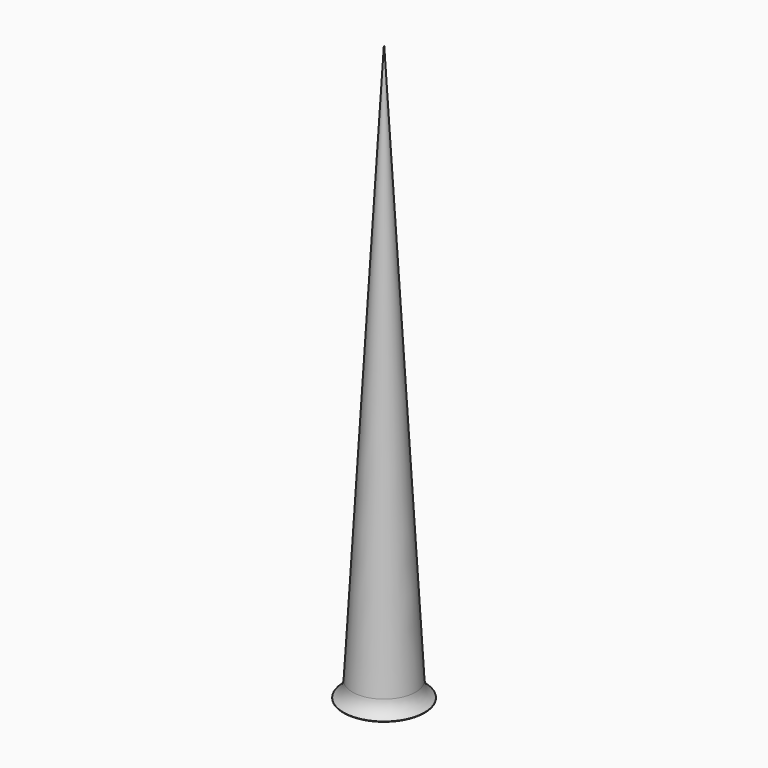
from build123d import *

# Parameters (mm, degrees)
F0_R     = 85
F2_R     = 0.5
F4_R     = 105.9677495378
F5_DEPTH = 1


# Not quite as in the source:
# - a fillet or chamfer that OpenCascade refuses, or shapes differently, is made with other operations: its cross-section is extruded or revolved along the edge and cut away or added


with BuildPart() as f3:
    # F0 (on Top) → F3 section 0
    with BuildSketch(Plane.XY):
        Circle(F0_R)
    # F2 (on offset) → F3 section 1
    with BuildSketch(Plane.XY.offset(1500)):
        Circle(F2_R)
    loft()

    # F4 (on Top) → F5 (join)
    with BuildSketch(Plane.XY):
        Circle(F4_R)
    extrude(amount=F5_DEPTH)

    # F6: fillet of radius 50 on 1 edges, made by hand


with BuildPart() as f6_tool2:
    # F6_s3 → F6_t4 (revolve)
    with BuildSketch(Plane.XZ):
        with BuildLine():
            ThreePointArc((105.9675361519, 0.9996616711), (89.555381413, 17.9202187852), (82.7192415892, 40.4797238448))
            Line((82.7192415892, 40.4797238448), (77.7270102291, 40.1984948115))
            ThreePointArc((77.7270102291, 40.1984948115), (78.8394224512, 20.458644138), (79.9514353065, 0.7187709667))
            Line((79.9514353065, 0.7187709667), (84.9436666667, -4.0001463701))
            ThreePointArc((84.9436666667, -4.0001463701), (95.4556014093, -4.0001463701), (103.300134248, -3.2295735796))
            Line((103.300134248, -3.2295735796), (105.9675361519, 0.9996616711))
        make_face()
    revolve(axis=Axis((0, 0, 1), (0, 0, 1)))

    split(bisect_by=Plane.XY, keep=Keep.TOP)


with BuildPart() as f3_1:
    add(f3.part)

    # F6_t1: union F6_tool2
    add(f6_tool2.part)


solid = f3_1.part
